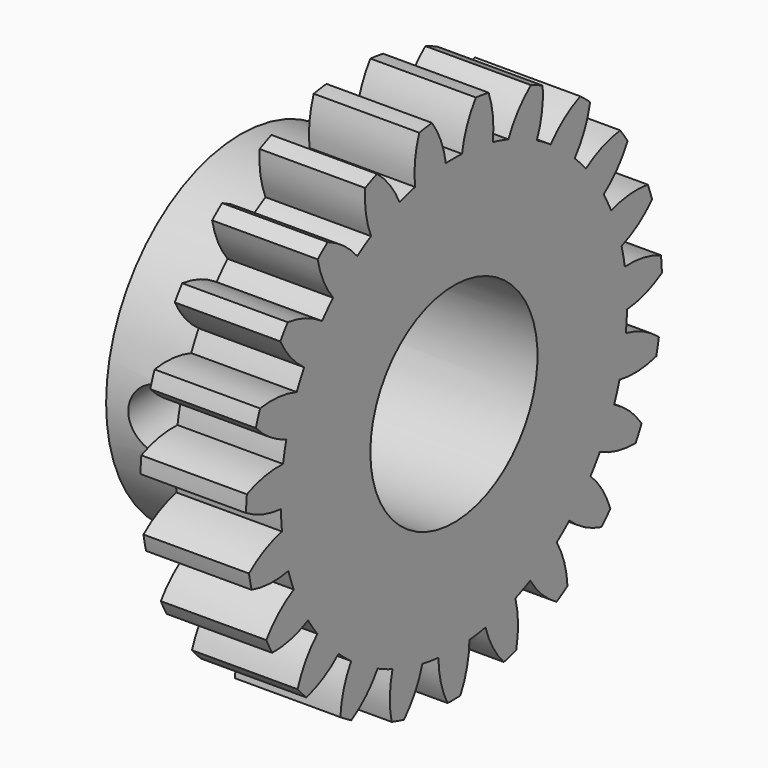
from build123d import *

# Parameters (mm, degrees)
F2_R            = 9.9
F3_DEPTH        = 25
F5_DEPTH        = 25
F5_COPIES_COUNT = 23
F7_R            = 2.95
F8_DEPTH        = 24.9


# Not quite as in the source:
# - a feature of the source that left no trace in its solid (it failed there, or was rolled back) is left out
# - a pattern or mirror of a feature is missing from the dataset's text; its kind, count and spacing are read off the source's solid


with BuildPart() as f1:
    # F0 (on Front) → F1 (revolve)
    with BuildSketch(Plane.XZ):
        Polygon((0, 15.95), (0, 0), (20.2, 0), (20.2, 24.65), (10.2, 24.65), (10.2, 15.95), align=None)
    revolve(axis=Axis((10.1, 0, 0), (-1, 0, 0)))

    # F2 (on face) → F3 (cut)
    with BuildSketch(Plane(origin=(0, 0, 0), x_dir=(0, -1, 0), z_dir=(-1, 0, 0))):
        Circle(F2_R)
    extrude(amount=-F3_DEPTH, mode=Mode.SUBTRACT)

    # F4 (on face) → F5 (cut)
    with BuildSketch(Plane.YZ.offset(20.2)):
        with BuildLine():
            ThreePointArc((0.9605272399, 20.4764837905), (1.5385061373, 22.5929437067), (2.6011700561, 24.5123726787))
            ThreePointArc((2.6011700561, 24.5123726787), (0, 24.65), (-2.6011700561, 24.5123726787))
            ThreePointArc((-2.6011700561, 24.5123726787), (-1.5385061373, 22.5929437067), (-0.9605272399, 20.4764837905))
            ThreePointArc((-0.9605272399, 20.4764837905), (0, 20.499), (0.9605272399, 20.4764837905))
        make_face()
        with BuildLine():
            ThreePointArc((2.6011700561, 24.5123726787), (2.7312798677, 24.6882080288), (2.8655332609, 24.8609004137))
            ThreePointArc((2.8655332609, 24.8609004137), (0, 25.0255), (-2.8655332609, 24.8609004137))
            ThreePointArc((-2.8655332609, 24.8609004137), (-2.7312798677, 24.6882080288), (-2.6011700561, 24.5123726787))
            ThreePointArc((-2.6011700561, 24.5123726787), (0, 24.65), (2.6011700561, 24.5123726787))
        make_face()
    f5 = extrude(amount=-F5_DEPTH, mode=Mode.SUBTRACT)

    # F5_copies: F5 ×23 about axis
    f5_copies_axis = Axis((0, 0, 0), (1, 0, 0))
    for i in range(1, F5_COPIES_COUNT):
        add(f5.rotate(f5_copies_axis, i * 360 / F5_COPIES_COUNT), mode=Mode.SUBTRACT)

    # F7 (on Front) → F8 (cut, symmetric)
    with BuildSketch(Plane.XZ):
        with Locations((5.05, 0)):
            Circle(F7_R)
    extrude(amount=F8_DEPTH, both=True, mode=Mode.SUBTRACT)


solid = f1.part
